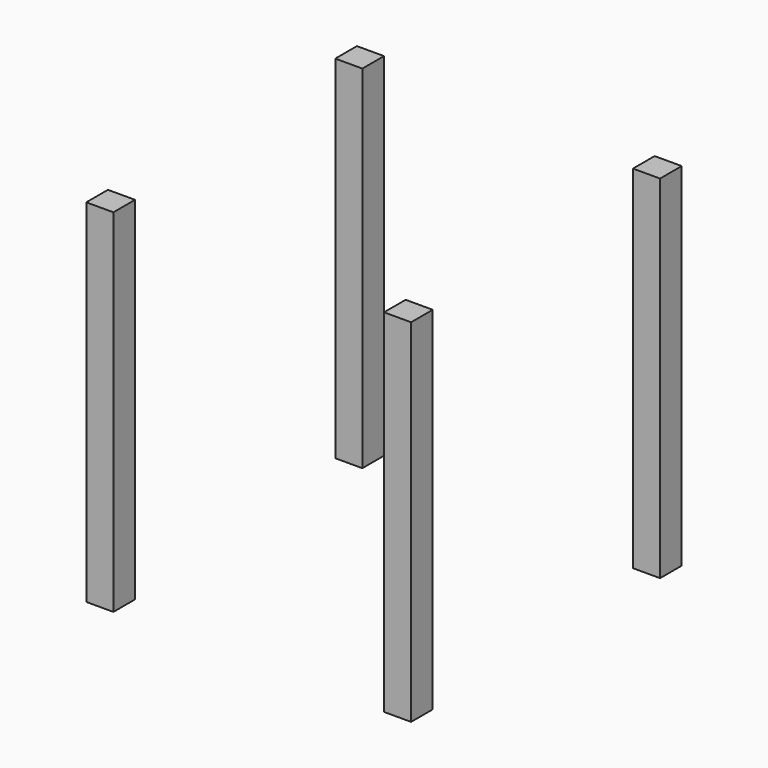
from build123d import *

# Parameters (mm, degrees)
F0_W     = 50.8
F0_H     = 50.8
F1_DEPTH = 330.2


# Not quite as in the source:
# - a feature names something its author has since deleted; it is built from what else it names


with BuildPart() as f1:
    # F0 (on Top) → F1 (new body, symmetric)
    with BuildSketch(Plane.XY):
        with Locations((-25.4, 355.3269766333)):
            Rectangle(F0_W, F0_H)
    extrude(amount=F1_DEPTH, both=True)


with BuildPart() as f1b:
    # F0 (on Top) → F1, piece 2 (new body, symmetric)
    with BuildSketch(Plane.XY):
        Polygon((-25.4, -203.4730233667), (-50.8, -203.4730233667), (-50.8, -254.2730233667), (0, -254.2730233667), (0, -203.4730233667), align=None)
    extrude(amount=F1_DEPTH, both=True)


with BuildPart() as f1c:
    # F0 (on Top) → F1, piece 3 (new body, symmetric)
    with BuildSketch(Plane.XY):
        Polygon((558.8, -254.2730233667), (558.8, -203.4730233667), (508, -203.4730233667), (508, -228.8730233667), (508, -254.2730233667), align=None)
    extrude(amount=F1_DEPTH, both=True)


with BuildPart() as f1d:
    # F0 (on Top) → F1, piece 4 (new body, symmetric)
    with BuildSketch(Plane.XY):
        with Locations((533.4, 355.3269766333)):
            Rectangle(F0_W, F0_H)
    extrude(amount=F1_DEPTH, both=True)


solid = Compound([f1.part, f1b.part, f1c.part, f1d.part])
